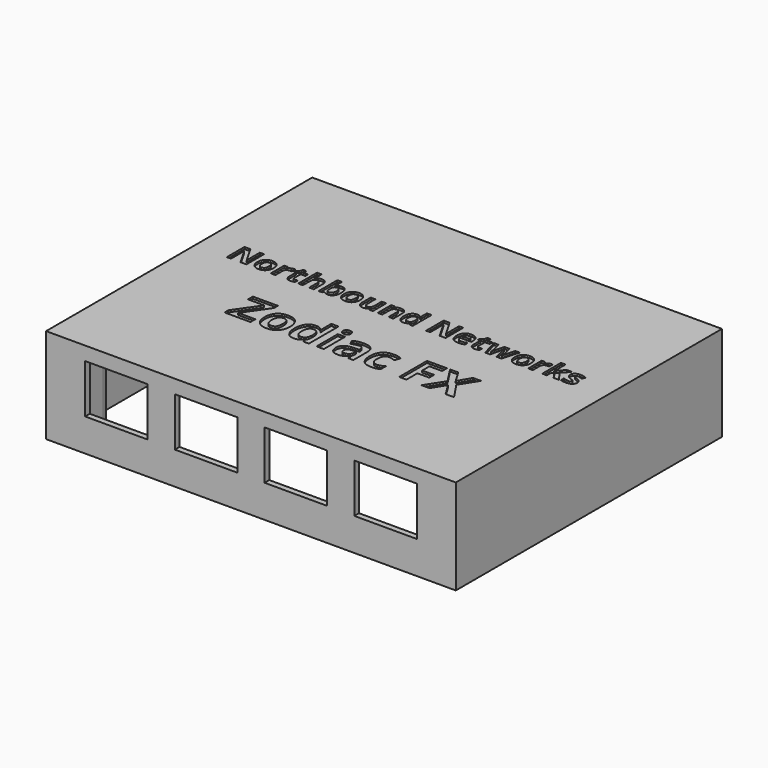
from build123d import *

# Parameters (mm, degrees)
F6_W            = 105
F6_H            = 85.25
F8_DEPTH        = 24.37
F6_W_2          = 10.5
F6_H_2          = 14
F9_DEPTH        = 1.5
F10_TEXT_SIZE   = 7.9311531842
F10_TEXT_SIZE_2 = 12.496421598
F11_DEPTH       = 0.5
F12_DEPTH       = 13.5
F7_W            = 16
F7_H            = 12.5
F13_DEPTH       = 42.625
F14_R           = 2
F15_DEPTH       = 42.625
F14_R_2         = 3.25
F16_DEPTH       = 27.125
F14_W           = 9
F14_H           = 3.5
F17_DEPTH       = 42.625


# Not quite as in the source:
# - Text() gives the source's letters only with a copy of the font that has no kerning and outlines rounded to 1/6400 em; it was checked with that copy


with BuildPart() as f8:
    # F6 (on Top) → F8 (new body, through all)
    with BuildSketch(Plane.XY):
        Rectangle(F6_W, F6_H)
        Polygon((43.25, 41.125), (51, 41.125), (51, 33.375), (51, -33.375), (51, -41.125), (43.25, -41.125), (-43.25, -41.125), (-51, -41.125), (-51, -33.375), (-51, 33.375), (-51, 41.125), (-43.25, 41.125), (28.3283032477, 41.125), (29.8283032477, 41.125), (40.3283032477, 41.125), (41.8283032477, 41.125), align=None, mode=Mode.SUBTRACT)
        with BuildLine():
            Line((-43.25, 35.875), (-43.25, 41.125))
            Line((-43.25, 41.125), (-51, 41.125))
            Line((-51, 41.125), (-51, 33.375))
            Line((-51, 33.375), (-45.75, 33.375))
            ThreePointArc((-45.75, 33.375), (-43.982233047, 34.107233047), (-43.25, 35.875))
        make_face()
        with BuildLine():
            Line((-51, -41.125), (-43.25, -41.125))
            Line((-43.25, -41.125), (-43.25, -35.875))
            ThreePointArc((-43.25, -35.875), (-43.982233047, -34.107233047), (-45.75, -33.375))
            Line((-45.75, -33.375), (-51, -33.375))
            Line((-51, -33.375), (-51, -41.125))
        make_face()
        with BuildLine():
            Line((51, -41.125), (51, -33.375))
            Line((51, -33.375), (45.75, -33.375))
            ThreePointArc((45.75, -33.375), (43.982233047, -34.107233047), (43.25, -35.875))
            Line((43.25, -35.875), (43.25, -41.125))
            Line((43.25, -41.125), (51, -41.125))
        make_face()
        with BuildLine():
            Line((51, 33.375), (51, 41.125))
            Line((51, 41.125), (43.25, 41.125))
            Line((43.25, 41.125), (43.25, 35.875))
            ThreePointArc((43.25, 35.875), (43.982233047, 34.107233047), (45.75, 33.375))
            Line((45.75, 33.375), (51, 33.375))
        make_face()
    extrude(amount=-F8_DEPTH)

    # F6 (on Top) → F9 (join)
    with BuildSketch(Plane.XY):
        with Locations((35.0783032477, 34.125)):
            Rectangle(F6_W_2, F6_H_2)
        Polygon((41.8283032477, 25.625), (41.8283032477, 41.125), (40.3283032477, 41.125), (40.3283032477, 27.125), (29.8283032477, 27.125), (29.8283032477, 41.125), (28.3283032477, 41.125), (28.3283032477, 25.625), align=None)
        with BuildLine():
            Line((43.25, 35.875), (43.25, 41.125))
            Line((43.25, 41.125), (41.8283032477, 41.125))
            Line((41.8283032477, 41.125), (41.8283032477, 25.625))
            Line((41.8283032477, 25.625), (28.3283032477, 25.625))
            Line((28.3283032477, 25.625), (28.3283032477, 41.125))
            Line((28.3283032477, 41.125), (-43.25, 41.125))
            Line((-43.25, 41.125), (-43.25, 35.875))
            ThreePointArc((-43.25, 35.875), (-43.982233047, 34.107233047), (-45.75, 33.375))
            Line((-45.75, 33.375), (-51, 33.375))
            Line((-51, 33.375), (-51, -33.375))
            Line((-51, -33.375), (-45.75, -33.375))
            ThreePointArc((-45.75, -33.375), (-43.982233047, -34.107233047), (-43.25, -35.875))
            Line((-43.25, -35.875), (-43.25, -41.125))
            Line((-43.25, -41.125), (43.25, -41.125))
            Line((43.25, -41.125), (43.25, -35.875))
            ThreePointArc((43.25, -35.875), (43.982233047, -34.107233047), (45.75, -33.375))
            Line((45.75, -33.375), (51, -33.375))
            Line((51, -33.375), (51, 33.375))
            Line((51, 33.375), (45.75, 33.375))
            ThreePointArc((45.75, 33.375), (43.982233047, 34.107233047), (43.25, 35.875))
        make_face()
    extrude(amount=-F9_DEPTH)

    # F10 (on Top) → F11 (cut)
    with BuildSketch(Plane.XY):
        with Locations((-45, 5)):
            Text('Northbound Networks', F10_TEXT_SIZE, font='Open Sans', font_style=FontStyle.BOLD, text_align=(TextAlign.LEFT, TextAlign.BOTTOM))
        with Locations((-29.9611470642, -13.9974235506)):
            Text('Zodiac FX', F10_TEXT_SIZE_2, font='Open Sans', font_style=FontStyle.BOLD, text_align=(TextAlign.LEFT, TextAlign.BOTTOM))
    extrude(amount=-F11_DEPTH, mode=Mode.SUBTRACT)

    # F6 (on Top) → F12 (join)
    with BuildSketch(Plane.XY):
        Polygon((41.8283032477, 25.625), (41.8283032477, 41.125), (40.3283032477, 41.125), (40.3283032477, 27.125), (29.8283032477, 27.125), (29.8283032477, 41.125), (28.3283032477, 41.125), (28.3283032477, 25.625), align=None)
    extrude(amount=-F12_DEPTH)

    # F7 (on Front) → F13 (cut, through all)
    with BuildSketch(Plane.XZ):
        with Locations((-34.5, -9.75)):
            Rectangle(F7_W, F7_H)
        with Locations((-11.5, -9.75)):
            Rectangle(F7_W, F7_H)
        with Locations((34.5, -9.75)):
            Rectangle(F7_W, F7_H)
        with Locations((11.5, -9.75)):
            Rectangle(F7_W, F7_H)
    extrude(amount=F13_DEPTH, mode=Mode.SUBTRACT)

    # F14 (on Front) → F15 (cut, through all)
    with BuildSketch(Plane.XZ):
        with Locations((35.0783032477, -8)):
            Circle(F14_R)
    extrude(amount=-F15_DEPTH, mode=Mode.SUBTRACT)

    # F14 (on Front) → F16 (cut, through all)
    with BuildSketch(Plane.XZ):
        with Locations((35.0783032477, -8)):
            Circle(F14_R_2)
        with Locations((35.0783032477, -8)):
            Circle(F14_R, mode=Mode.SUBTRACT)
    extrude(amount=-F16_DEPTH, mode=Mode.SUBTRACT)

    # F14 (on Front) → F17 (cut, through all)
    with BuildSketch(Plane.XZ):
        with Locations((-35.5, -14.25)):
            Rectangle(F14_W, F14_H)
    extrude(amount=-F17_DEPTH, mode=Mode.SUBTRACT)


solid = f8.part
